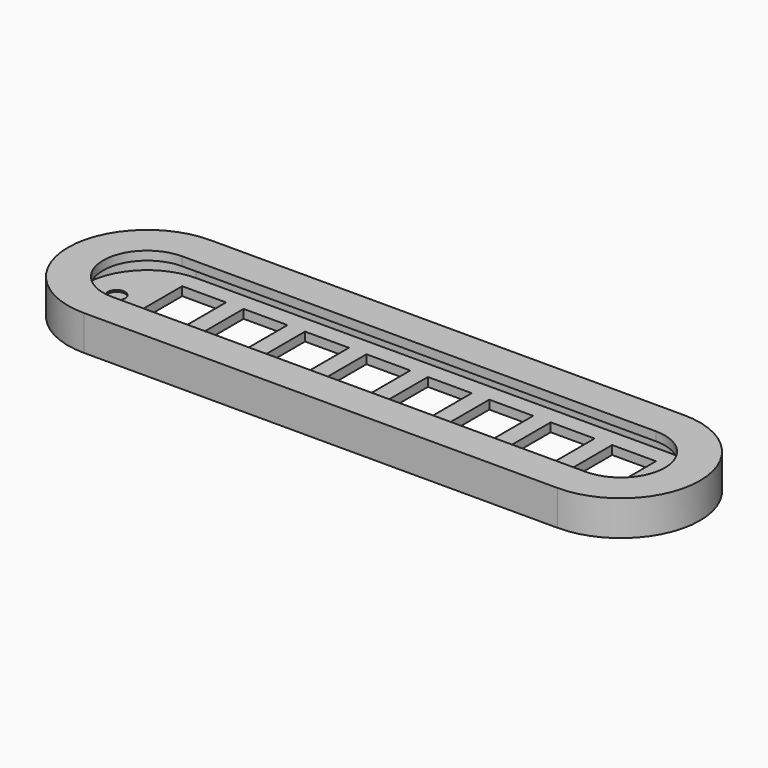
from build123d import *

# Parameters (mm, degrees)
F1_DEPTH  = 0.5
F2_W      = 2.5
F2_H      = 5
F3_DEPTH  = 0.501
F4_DEPTH  = 1
F6_DEPTH  = 0.5
F8_DEPTH  = 0.1
F10_DEPTH = 0.25


# Not quite as in the source:
# - a feature names something its author has since deleted; it is built from what else it names


with BuildPart() as f1:
    # F0 (on Top) → F1 (new body)
    with BuildSketch(Plane.XY):
        with BuildLine():
            Line((0, 4.5), (-13.5, 4.5))
            ThreePointArc((-13.5, 4.5), (-18, 0), (-13.5, -4.5))
            Line((-13.5, -4.5), (0, -4.5))
            Line((0, -4.5), (13.5, -4.5))
            ThreePointArc((13.5, -4.5), (18, 0), (13.5, 4.5))
            Line((13.5, 4.5), (0, 4.5))
        make_face()
    extrude(amount=F1_DEPTH)

    # F2 (on face) → F3 (cut, through all)
    with BuildSketch(Plane.XY.offset(0.5)):
        with Locations((-12.25, 0)):
            Rectangle(F2_W, F2_H)
        with Locations((-5.25, 0)):
            Rectangle(F2_W, F2_H)
        with Locations((-1.75, 0)):
            Rectangle(F2_W, F2_H)
        with Locations((-8.75, 0)):
            Rectangle(F2_W, F2_H)
        with Locations((1.75, 0)):
            Rectangle(F2_W, F2_H)
        with Locations((5.25, 0)):
            Rectangle(F2_W, F2_H)
        with Locations((8.75, 0)):
            Rectangle(F2_W, F2_H)
        with Locations((12.25, 0)):
            Rectangle(F2_W, F2_H)
    extrude(amount=-F3_DEPTH, mode=Mode.SUBTRACT)

    # F2 (on face) → F4 (join)
    with BuildSketch(Plane.XY.offset(0.5)):
        with BuildLine():
            Line((0, 4.5), (-13.5, 4.5))
            ThreePointArc((-13.5, 4.5), (-18, 0), (-13.5, -4.5))
            Line((-13.5, -4.5), (0, -4.5))
            Line((0, -4.5), (13.5, -4.5))
            ThreePointArc((13.5, -4.5), (18, 0), (13.5, 4.5))
            Line((13.5, 4.5), (0, 4.5))
        make_face()
        with BuildLine():
            ThreePointArc((-13.5, -3.5), (-17, 0), (-13.5, 3.5))
            Line((-13.5, 3.5), (0, 3.5))
            Line((0, 3.5), (13.5, 3.5))
            ThreePointArc((13.5, 3.5), (17, 0), (13.5, -3.5))
            Line((13.5, -3.5), (0, -3.5))
            Line((0, -3.5), (-13.5, -3.5))
        make_face(mode=Mode.SUBTRACT)
    extrude(amount=F4_DEPTH)

    # F5 (on face) → F6 (join)
    with BuildSketch(Plane.XY.offset(1.5)):
        with BuildLine():
            Line((0, 4.5), (-13.5, 4.5))
            ThreePointArc((-13.5, 4.5), (-18, 0), (-13.5, -4.5))
            Line((-13.5, -4.5), (0, -4.5))
            Line((0, -4.5), (13.5, -4.5))
            ThreePointArc((13.5, -4.5), (18, 0), (13.5, 4.5))
            Line((13.5, 4.5), (0, 4.5))
        make_face()
        with BuildLine():
            Line((13.5, -3.5), (-13.5, -3.5))
            ThreePointArc((-13.5, -3.5), (-17, 0), (-13.5, 3.5))
            Line((-13.5, 3.5), (13.5, 3.5))
            ThreePointArc((13.5, 3.5), (17, 0), (13.5, -3.5))
        make_face(mode=Mode.SUBTRACT)
        with BuildLine():
            ThreePointArc((-13.5, 3.5), (-17, 0), (-13.5, -3.5))
            Line((-13.5, -3.5), (13.5, -3.5))
            ThreePointArc((13.5, -3.5), (17, 0), (13.5, 3.5))
            Line((13.5, 3.5), (-13.5, 3.5))
        make_face()
        with BuildLine():
            ThreePointArc((-13.5, -2.5), (-16, 0), (-13.5, 2.5))
            Line((-13.5, 2.5), (0, 2.5))
            Line((0, 2.5), (13.5, 2.5))
            ThreePointArc((13.5, 2.5), (16, 0), (13.5, -2.5))
            Line((13.5, -2.5), (0, -2.5))
            Line((0, -2.5), (-13.5, -2.5))
        make_face(mode=Mode.SUBTRACT)
    extrude(amount=F6_DEPTH)

    # F7 (on face) → F8 (cut)
    with BuildSketch(Plane.XY.offset(0.5)):
        with BuildLine():
            ThreePointArc((-15.75, 0), (-15.25, -0.5), (-14.75, 0))
            ThreePointArc((-14.75, 0), (-15.25, 0.5), (-15.75, 0))
        make_face()
    extrude(amount=-F8_DEPTH, mode=Mode.SUBTRACT)

    # F9 (on face) → F10 (cut)
    with BuildSketch(Plane(origin=(0, 0, 0), x_dir=(1, 0, 0), z_dir=(0, 0, -1))):
        with BuildLine():
            ThreePointArc((-15.75, 0), (-15.25, -0.5), (-14.75, 0))
            ThreePointArc((-14.75, 0), (-15.25, 0.5), (-15.75, 0))
        make_face()
    extrude(amount=-F10_DEPTH, mode=Mode.SUBTRACT)


solid = f1.part
